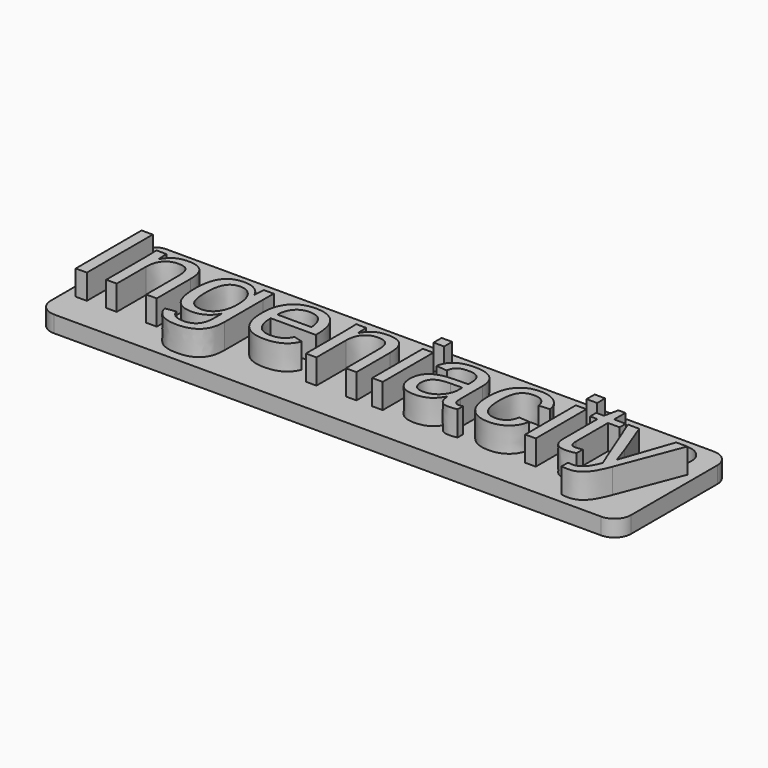
from build123d import *

# Parameters (mm, degrees)
F0_TEXT_SIZE = 14.4390369678
F1_DEPTH     = 3
F0_W         = 1.2701840333
F0_H         = 7.6278724981
F0_W_2       = 1.3468914172
F0_H_2       = 9.9336062139
F0_H_3       = 1.2137815451
F0_R         = 2
F2_DEPTH     = 2
F3_DEPTH     = 2


# Not quite as in the source:
# - Text() gives the source's letters only with a copy of the font that has no kerning and outlines rounded to 1/6400 em; it was checked with that copy


with BuildPart() as f1:
    # F0 (on Top) → F1 (new body)
    with BuildSketch(Plane.XY):
        with Locations((0, 4.1038933832)):
            Text('Ingeniacity', F0_TEXT_SIZE, font='Arimo', text_align=(TextAlign.LEFT, TextAlign.BOTTOM))
    extrude(amount=F1_DEPTH)


with BuildPart() as f2:
    # F0 (on Top) → F2 (new body)
    with BuildSketch(Plane.XY):
        with BuildLine():
            ThreePointArc((0, 2), (0.5857864376, 0.5857864376), (2, 0))
            Line((2, 0), (68, 0))
            ThreePointArc((68, 0), (69.4142135624, 0.5857864376), (70, 2))
            Line((70, 2), (70, 15))
            ThreePointArc((70, 15), (69.4142135624, 16.4142135624), (68, 17))
            Line((68, 17), (2, 17))
            ThreePointArc((2, 17), (0.5857864376, 16.4142135624), (0, 15))
            Line((0, 15), (0, 2))
        make_face()
        with BuildLine():
            Line((11.1045218681, 4.1038933832), (9.8275695362, 4.1038933832))
            Line((9.8275695362, 4.1038933832), (9.8275695362, 8.9409707674))
            add(Edge.make_bspline(
                [(9.8275695362, 8.9409707674), (9.8275695362, 9.6945080092), (9.6797950172, 10.1107583717)],
                knots=[0, 0, 0, 1, 1, 1], degree=2))
            add(Edge.make_bspline(
                [(9.6797950172, 10.1107583717), (9.5320204983, 10.5270087343), (9.2071421665, 10.709752796)],
                knots=[0, 0, 0, 1, 1, 1], degree=2))
            add(Edge.make_bspline(
                [(9.2071421665, 10.709752796), (8.8822638347, 10.8924968576), (8.2550681664, 10.8924968576)],
                knots=[0, 0, 0, 1, 1, 1], degree=2))
            add(Edge.make_bspline(
                [(8.2550681664, 10.8924968576), (7.3390917588, 10.8924968576), (6.8100364199, 10.2653011893)],
                knots=[0, 0, 0, 1, 1, 1], degree=2))
            add(Edge.make_bspline(
                [(6.8100364199, 10.2653011893), (6.280981081, 9.638105521), (6.280981081, 8.523592355)],
                knots=[0, 0, 0, 1, 1, 1], degree=2))
            Line((6.280981081, 8.523592355), (6.280981081, 4.1038933832))
            Line((6.280981081, 4.1038933832), (5.0130531473, 4.1038933832))
            Line((5.0130531473, 4.1038933832), (5.0130531473, 10.1028620234))
            add(Edge.make_bspline(
                [(5.0130531473, 10.1028620234), (5.0130531473, 11.4362168434), (4.9701872563, 11.7317658813)],
                knots=[0, 0, 0, 1, 1, 1], degree=2))
            Line((4.9701872563, 11.7317658813), (6.1681761047, 11.7317658813))
            add(Edge.make_bspline(
                [(6.1681761047, 11.7317658813), (6.1749444033, 11.6979243884), (6.1828407516, 11.5422535211)],
                knots=[0, 0, 0, 1, 1, 1], degree=2))
            add(Edge.make_bspline(
                [(6.1828407516, 11.5422535211), (6.1907370999, 11.3865826538), (6.2008895478, 11.185789796)],
                knots=[0, 0, 0, 1, 1, 1], degree=2))
            add(Edge.make_bspline(
                [(6.2008895478, 11.185789796), (6.2110419957, 10.9849969382), (6.2245785928, 10.4277403552)],
                knots=[0, 0, 0, 1, 1, 1], degree=2))
            Line((6.2245785928, 10.4277403552), (6.2471395881, 10.4277403552))
            add(Edge.make_bspline(
                [(6.2471395881, 10.4277403552), (6.6825667967, 11.2173751894), (7.2578721758, 11.5456376704)],
                knots=[0, 0, 0, 1, 1, 1], degree=2))
            add(Edge.make_bspline(
                [(7.2578721758, 11.5456376704), (7.833177555, 11.8739001515), (8.6859831759, 11.8739001515)],
                knots=[0, 0, 0, 1, 1, 1], degree=2))
            add(Edge.make_bspline(
                [(8.6859831759, 11.8739001515), (9.9403745125, 11.8739001515), (10.5224481903, 11.2500886325)],
                knots=[0, 0, 0, 1, 1, 1], degree=2))
            add(Edge.make_bspline(
                [(10.5224481903, 11.2500886325), (11.1045218681, 10.6262771135), (11.1045218681, 9.1868856158)],
                knots=[0, 0, 0, 1, 1, 1], degree=2))
            Line((11.1045218681, 9.1868856158), (11.1045218681, 4.1038933832))
        make_face(mode=Mode.SUBTRACT)
        with BuildLine():
            add(Edge.make_bspline(
                [(19.0978824894, 4.3227350372), (19.0978824894, 1.1077932124), (15.9055016598, 1.1077932124)],
                knots=[0, 0, 0, 1, 1, 1], degree=2))
            add(Edge.make_bspline(
                [(15.9055016598, 1.1077932124), (14.6556225223, 1.1077932124), (13.9156218777, 1.5973668096)],
                knots=[0, 0, 0, 1, 1, 1], degree=2))
            add(Edge.make_bspline(
                [(13.9156218777, 1.5973668096), (13.1756212331, 2.0869404067), (12.9635478777, 2.9893802172)],
                knots=[0, 0, 0, 1, 1, 1], degree=2))
            Line((12.9635478777, 2.9893802172), (14.2405002095, 3.1721242789))
            add(Edge.make_bspline(
                [(14.2405002095, 3.1721242789), (14.366841783, 2.6441969897), (14.8011409418, 2.3588003997)],
                knots=[0, 0, 0, 1, 1, 1], degree=2))
            add(Edge.make_bspline(
                [(14.8011409418, 2.3588003997), (15.2354401006, 2.0734038096), (15.9393431527, 2.0734038096)],
                knots=[0, 0, 0, 1, 1, 1], degree=2))
            add(Edge.make_bspline(
                [(15.9393431527, 2.0734038096), (17.8367228543, 2.0734038096), (17.8367228543, 4.2934057434)],
                knots=[0, 0, 0, 1, 1, 1], degree=2))
            Line((17.8367228543, 4.2934057434), (17.8367228543, 5.5207238856))
            Line((17.8367228543, 5.5207238856), (17.8231862571, 5.5207238856))
            add(Edge.make_bspline(
                [(17.8231862571, 5.5207238856), (17.4622103329, 4.7874915396), (16.8350146646, 4.4174912173)],
                knots=[0, 0, 0, 1, 1, 1], degree=2))
            add(Edge.make_bspline(
                [(16.8350146646, 4.4174912173), (16.2078189964, 4.047490895), (15.3685499726, 4.047490895)],
                knots=[0, 0, 0, 1, 1, 1], degree=2))
            add(Edge.make_bspline(
                [(15.3685499726, 4.047490895), (13.9652560673, 4.047490895), (13.3064750056, 4.9781319496)],
                knots=[0, 0, 0, 1, 1, 1], degree=2))
            add(Edge.make_bspline(
                [(13.3064750056, 4.9781319496), (12.647693944, 5.9087730042), (12.647693944, 7.9031649853)],
                knots=[0, 0, 0, 1, 1, 1], degree=2))
            add(Edge.make_bspline(
                [(12.647693944, 7.9031649853), (12.647693944, 9.9268862604), (13.3561091952, 10.8891127083)],
                knots=[0, 0, 0, 1, 1, 1], degree=2))
            add(Edge.make_bspline(
                [(13.3561091952, 10.8891127083), (14.0645244464, 11.8513391562), (15.5106842428, 11.8513391562)],
                knots=[0, 0, 0, 1, 1, 1], degree=2))
            add(Edge.make_bspline(
                [(15.5106842428, 11.8513391562), (16.3206239727, 11.8513391562), (16.9162342476, 11.4813388339)],
                knots=[0, 0, 0, 1, 1, 1], degree=2))
            add(Edge.make_bspline(
                [(16.9162342476, 11.4813388339), (17.5118445225, 11.1113385116), (17.8367228543, 10.4277403552)],
                knots=[0, 0, 0, 1, 1, 1], degree=2))
            Line((17.8367228543, 10.4277403552), (17.8502594514, 10.4277403552))
            add(Edge.make_bspline(
                [(17.8502594514, 10.4277403552), (17.8502594514, 10.6398137106), (17.8784606955, 11.1609727012)],
                knots=[0, 0, 0, 1, 1, 1], degree=2))
            add(Edge.make_bspline(
                [(17.8784606955, 11.1609727012), (17.9066619396, 11.6821316918), (17.9359912334, 11.7317658813)],
                knots=[0, 0, 0, 1, 1, 1], degree=2))
            Line((17.9359912334, 11.7317658813), (19.1407483804, 11.7317658813))
            add(Edge.make_bspline(
                [(19.1407483804, 11.7317658813), (19.0978824894, 11.3527411609), (19.0978824894, 10.152496213)],
                knots=[0, 0, 0, 1, 1, 1], degree=2))
            Line((19.0978824894, 10.152496213), (19.0978824894, 4.3227350372))
        make_face(mode=Mode.SUBTRACT)
        with BuildLine():
            Line((27.4589873336, 7.6504818384), (22.0172752764, 7.6504818384))
            add(Edge.make_bspline(
                [(22.0172752764, 7.6504818384), (22.0172752764, 6.3396880137), (22.5598672124, 5.6267605634)],
                knots=[0, 0, 0, 1, 1, 1], degree=2))
            add(Edge.make_bspline(
                [(22.5598672124, 5.6267605634), (23.1024591485, 4.9138331131), (24.1447771296, 4.9138331131)],
                knots=[0, 0, 0, 1, 1, 1], degree=2))
            add(Edge.make_bspline(
                [(24.1447771296, 4.9138331131), (24.9705095562, 4.9138331131), (25.4679795017, 5.2454797434)],
                knots=[0, 0, 0, 1, 1, 1], degree=2))
            add(Edge.make_bspline(
                [(25.4679795017, 5.2454797434), (25.9654494473, 5.5771263738), (26.1414252103, 6.0847487672)],
                knots=[0, 0, 0, 1, 1, 1], degree=2))
            Line((26.1414252103, 6.0847487672), (27.2536822767, 5.7688948335))
            add(Edge.make_bspline(
                [(27.2536822767, 5.7688948335), (26.5700841203, 3.961759113), (24.1447771296, 3.961759113)],
                knots=[0, 0, 0, 1, 1, 1], degree=2))
            add(Edge.make_bspline(
                [(24.1447771296, 3.961759113), (22.4527024849, 3.961759113), (21.5683114707, 4.9702356013)],
                knots=[0, 0, 0, 1, 1, 1], degree=2))
            add(Edge.make_bspline(
                [(21.5683114707, 4.9702356013), (20.6839204564, 5.9787120895), (20.6839204564, 7.9685918716)],
                knots=[0, 0, 0, 1, 1, 1], degree=2))
            add(Edge.make_bspline(
                [(20.6839204564, 7.9685918716), (20.6839204564, 9.856947175), (21.5683114707, 10.8654236633)],
                knots=[0, 0, 0, 1, 1, 1], degree=2))
            add(Edge.make_bspline(
                [(21.5683114707, 10.8654236633), (22.4527024849, 11.8739001515), (24.09514294, 11.8739001515)],
                knots=[0, 0, 0, 1, 1, 1], degree=2))
            add(Edge.make_bspline(
                [(24.09514294, 11.8739001515), (27.4589873336, 11.8739001515), (27.4589873336, 7.8196893029)],
                knots=[0, 0, 0, 1, 1, 1], degree=2))
            Line((27.4589873336, 7.8196893029), (27.4589873336, 7.6504818384))
        make_face(mode=Mode.SUBTRACT)
        with BuildLine():
            Line((35.1928965095, 4.1038933832), (33.9159441777, 4.1038933832))
            Line((33.9159441777, 4.1038933832), (33.9159441777, 8.9409707674))
            add(Edge.make_bspline(
                [(33.9159441777, 8.9409707674), (33.9159441777, 9.6945080092), (33.7681696587, 10.1107583717)],
                knots=[0, 0, 0, 1, 1, 1], degree=2))
            add(Edge.make_bspline(
                [(33.7681696587, 10.1107583717), (33.6203951397, 10.5270087343), (33.2955168079, 10.709752796)],
                knots=[0, 0, 0, 1, 1, 1], degree=2))
            add(Edge.make_bspline(
                [(33.2955168079, 10.709752796), (32.9706384762, 10.8924968576), (32.3434428079, 10.8924968576)],
                knots=[0, 0, 0, 1, 1, 1], degree=2))
            add(Edge.make_bspline(
                [(32.3434428079, 10.8924968576), (31.4274664002, 10.8924968576), (30.8984110613, 10.2653011893)],
                knots=[0, 0, 0, 1, 1, 1], degree=2))
            add(Edge.make_bspline(
                [(30.8984110613, 10.2653011893), (30.3693557224, 9.638105521), (30.3693557224, 8.523592355)],
                knots=[0, 0, 0, 1, 1, 1], degree=2))
            Line((30.3693557224, 8.523592355), (30.3693557224, 4.1038933832))
            Line((30.3693557224, 4.1038933832), (29.1014277887, 4.1038933832))
            Line((29.1014277887, 4.1038933832), (29.1014277887, 10.1028620234))
            add(Edge.make_bspline(
                [(29.1014277887, 10.1028620234), (29.1014277887, 11.4362168434), (29.0585618977, 11.7317658813)],
                knots=[0, 0, 0, 1, 1, 1], degree=2))
            Line((29.0585618977, 11.7317658813), (30.2565507461, 11.7317658813))
            add(Edge.make_bspline(
                [(30.2565507461, 11.7317658813), (30.2633190447, 11.6979243884), (30.271215393, 11.5422535211)],
                knots=[0, 0, 0, 1, 1, 1], degree=2))
            add(Edge.make_bspline(
                [(30.271215393, 11.5422535211), (30.2791117414, 11.3865826538), (30.2892641893, 11.185789796)],
                knots=[0, 0, 0, 1, 1, 1], degree=2))
            add(Edge.make_bspline(
                [(30.2892641893, 11.185789796), (30.2994166371, 10.9849969382), (30.3129532343, 10.4277403552)],
                knots=[0, 0, 0, 1, 1, 1], degree=2))
            Line((30.3129532343, 10.4277403552), (30.3355142295, 10.4277403552))
            add(Edge.make_bspline(
                [(30.3355142295, 10.4277403552), (30.7709414381, 11.2173751894), (31.3462468173, 11.5456376704)],
                knots=[0, 0, 0, 1, 1, 1], degree=2))
            add(Edge.make_bspline(
                [(31.3462468173, 11.5456376704), (31.9215521965, 11.8739001515), (32.7743578174, 11.8739001515)],
                knots=[0, 0, 0, 1, 1, 1], degree=2))
            add(Edge.make_bspline(
                [(32.7743578174, 11.8739001515), (34.028749154, 11.8739001515), (34.6108228317, 11.2500886325)],
                knots=[0, 0, 0, 1, 1, 1], degree=2))
            add(Edge.make_bspline(
                [(34.6108228317, 11.2500886325), (35.1928965095, 10.6262771135), (35.1928965095, 9.1868856158)],
                knots=[0, 0, 0, 1, 1, 1], degree=2))
            Line((35.1928965095, 9.1868856158), (35.1928965095, 4.1038933832))
        make_face(mode=Mode.SUBTRACT)
        with Locations((37.7298804267, 7.9178296323)):
            Rectangle(F0_W, F0_H, mode=Mode.SUBTRACT)
        with BuildLine():
            add(Edge.make_bspline(
                [(43.8247332968, 4.3249911368), (43.1794888323, 3.961759113), (42.2567441261, 3.961759113)],
                knots=[0, 0, 0, 1, 1, 1], degree=2))
            add(Edge.make_bspline(
                [(42.2567441261, 3.961759113), (41.1061333677, 3.961759113), (40.528571889, 4.5686498856)],
                knots=[0, 0, 0, 1, 1, 1], degree=2))
            add(Edge.make_bspline(
                [(40.528571889, 4.5686498856), (39.9510104103, 5.1755406581), (39.9510104103, 6.2336513359)],
                knots=[0, 0, 0, 1, 1, 1], degree=2))
            add(Edge.make_bspline(
                [(39.9510104103, 6.2336513359), (39.9510104103, 7.4181035872), (40.7304927966, 8.0520675541)],
                knots=[0, 0, 0, 1, 1, 1], degree=2))
            add(Edge.make_bspline(
                [(40.7304927966, 8.0520675541), (41.5099751829, 8.6860315209), (43.242659619, 8.7288974119)],
                knots=[0, 0, 0, 1, 1, 1], degree=2))
            Line((43.242659619, 8.7288974119), (44.957295259, 8.7582267058))
            Line((44.957295259, 8.7582267058), (44.957295259, 9.1733490186))
            add(Edge.make_bspline(
                [(44.957295259, 9.1733490186), (44.957295259, 10.1028620234), (44.5624778419, 10.5055757888)],
                knots=[0, 0, 0, 1, 1, 1], degree=2))
            add(Edge.make_bspline(
                [(44.5624778419, 10.5055757888), (44.1676604248, 10.9082895543), (43.3216231025, 10.9082895543)],
                knots=[0, 0, 0, 1, 1, 1], degree=2))
            add(Edge.make_bspline(
                [(43.3216231025, 10.9082895543), (42.4688174815, 10.9082895543), (42.080768363, 10.6183807651)],
                knots=[0, 0, 0, 1, 1, 1], degree=2))
            add(Edge.make_bspline(
                [(42.080768363, 10.6183807651), (41.6927192445, 10.328471976), (41.6137557611, 9.6945080092)],
                knots=[0, 0, 0, 1, 1, 1], degree=2))
            Line((41.6137557611, 9.6945080092), (40.2894253392, 9.814081284))
            add(Edge.make_bspline(
                [(40.2894253392, 9.814081284), (40.614303671, 11.8739001515), (43.3486962968, 11.8739001515)],
                knots=[0, 0, 0, 1, 1, 1], degree=2))
            add(Edge.make_bspline(
                [(43.3486962968, 11.8739001515), (44.7880877945, 11.8739001515), (45.5134237922, 11.2139910401)],
                knots=[0, 0, 0, 1, 1, 1], degree=2))
            add(Edge.make_bspline(
                [(45.5134237922, 11.2139910401), (46.2387597899, 10.5540819286), (46.2387597899, 9.3064588906)],
                knots=[0, 0, 0, 1, 1, 1], degree=2))
            Line((46.2387597899, 9.3064588906), (46.2387597899, 6.0215779805))
            add(Edge.make_bspline(
                [(46.2387597899, 6.0215779805), (46.2387597899, 5.4575530989), (46.3876623586, 5.1721565088)],
                knots=[0, 0, 0, 1, 1, 1], degree=2))
            add(Edge.make_bspline(
                [(46.3876623586, 5.1721565088), (46.5365649273, 4.8867599188), (46.9516872401, 4.8867599188)],
                knots=[0, 0, 0, 1, 1, 1], degree=2))
            add(Edge.make_bspline(
                [(46.9516872401, 4.8867599188), (47.1344313018, 4.8867599188), (47.366809553, 4.9363941084)],
                knots=[0, 0, 0, 1, 1, 1], degree=2))
            Line((47.366809553, 4.9363941084), (47.366809553, 4.1467592742))
            add(Edge.make_bspline(
                [(47.366809553, 4.1467592742), (46.8885164534, 4.0339542979), (46.3876623586, 4.0339542979)],
                knots=[0, 0, 0, 1, 1, 1], degree=2))
            add(Edge.make_bspline(
                [(46.3876623586, 4.0339542979), (45.6837593064, 4.0339542979), (45.3622651239, 4.4039546202)],
                knots=[0, 0, 0, 1, 1, 1], degree=2))
            add(Edge.make_bspline(
                [(45.3622651239, 4.4039546202), (45.0407709414, 4.7739549425), (44.9979050504, 5.5635897766)],
                knots=[0, 0, 0, 1, 1, 1], degree=2))
            Line((44.9979050504, 5.5635897766), (44.957295259, 5.5635897766))
            add(Edge.make_bspline(
                [(44.957295259, 5.5635897766), (44.4699777613, 4.6882231605), (43.8247332968, 4.3249911368)],
                knots=[0, 0, 0, 1, 1, 1], degree=2))
        make_face(mode=Mode.SUBTRACT)
        with BuildLine():
            add(Edge.make_bspline(
                [(49.7560189512, 10.2088987011), (49.304799046, 9.5388371418), (49.304799046, 7.9527991749)],
                knots=[0, 0, 0, 1, 1, 1], degree=2))
            add(Edge.make_bspline(
                [(49.304799046, 7.9527991749), (49.304799046, 6.4299319947), (49.7842201953, 5.6966996487)],
                knots=[0, 0, 0, 1, 1, 1], degree=2))
            add(Edge.make_bspline(
                [(49.7842201953, 5.6966996487), (50.2636413446, 4.9634673027), (51.2315080414, 4.9634673027)],
                knots=[0, 0, 0, 1, 1, 1], degree=2))
            add(Edge.make_bspline(
                [(51.2315080414, 4.9634673027), (51.9083378992, 4.9634673027), (52.3629419538, 5.3300834757)],
                knots=[0, 0, 0, 1, 1, 1], degree=2))
            add(Edge.make_bspline(
                [(52.3629419538, 5.3300834757), (52.8175460083, 5.6966996487), (52.923582686, 6.4592612886)],
                knots=[0, 0, 0, 1, 1, 1], degree=2))
            Line((52.923582686, 6.4592612886), (54.2050472169, 6.3735295066))
            add(Edge.make_bspline(
                [(54.2050472169, 6.3735295066), (54.0584007477, 5.2748090373), (53.2687659136, 4.6182840752)],
                knots=[0, 0, 0, 1, 1, 1], degree=2))
            add(Edge.make_bspline(
                [(53.2687659136, 4.6182840752), (52.4791310794, 3.961759113), (51.2653495343, 3.961759113)],
                knots=[0, 0, 0, 1, 1, 1], degree=2))
            add(Edge.make_bspline(
                [(51.2653495343, 3.961759113), (49.6657749702, 3.961759113), (48.8231217971, 4.9736197505)],
                knots=[0, 0, 0, 1, 1, 1], degree=2))
            add(Edge.make_bspline(
                [(48.8231217971, 4.9736197505), (47.9804686241, 5.985480388), (47.9804686241, 7.9257259806)],
                knots=[0, 0, 0, 1, 1, 1], degree=2))
            add(Edge.make_bspline(
                [(47.9804686241, 7.9257259806), (47.9804686241, 9.8501788765), (48.8265059464, 10.862039514)],
                knots=[0, 0, 0, 1, 1, 1], degree=2))
            add(Edge.make_bspline(
                [(48.8265059464, 10.862039514), (49.6725432688, 11.8739001515), (51.2518129371, 11.8739001515)],
                knots=[0, 0, 0, 1, 1, 1], degree=2))
            add(Edge.make_bspline(
                [(51.2518129371, 11.8739001515), (52.4227285912, 11.8739001515), (53.1943146292, 11.2670093789)],
                knots=[0, 0, 0, 1, 1, 1], degree=2))
            add(Edge.make_bspline(
                [(53.1943146292, 11.2670093789), (53.9659006672, 10.6601186064), (54.1644374255, 9.59523963)],
                knots=[0, 0, 0, 1, 1, 1], degree=2))
            Line((54.1644374255, 9.59523963), (52.8581557998, 9.4982273504))
            add(Edge.make_bspline(
                [(52.8581557998, 9.4982273504), (52.7611435202, 10.1321913172), (52.3584297547, 10.5055757888)],
                knots=[0, 0, 0, 1, 1, 1], degree=2))
            add(Edge.make_bspline(
                [(52.3584297547, 10.5055757888), (51.9557159893, 10.8789602604), (51.2157153447, 10.8789602604)],
                knots=[0, 0, 0, 1, 1, 1], degree=2))
            add(Edge.make_bspline(
                [(51.2157153447, 10.8789602604), (50.2072388565, 10.8789602604), (49.7560189512, 10.2088987011)],
                knots=[0, 0, 0, 1, 1, 1], degree=2))
        make_face(mode=Mode.SUBTRACT)
        with Locations((56.1870306507, 7.9178296323)):
            Rectangle(F0_W, F0_H, mode=Mode.SUBTRACT)
        with BuildLine():
            add(Edge.make_bspline(
                [(64.2774035517, 1.399958101), (63.7799336062, 1.1077932124), (63.1527379379, 1.1077932124)],
                knots=[0, 0, 0, 1, 1, 1], degree=2))
            add(Edge.make_bspline(
                [(63.1527379379, 1.1077932124), (62.6315789474, 1.1077932124), (62.2773713218, 1.1845005963)],
                knots=[0, 0, 0, 1, 1, 1], degree=2))
            Line((62.2773713218, 1.1845005963), (62.2773713218, 2.1365745963))
            add(Edge.make_bspline(
                [(62.2773713218, 2.1365745963), (62.5458471654, 2.0937087053), (62.8707254971, 2.0937087053)],
                knots=[0, 0, 0, 1, 1, 1], degree=2))
            add(Edge.make_bspline(
                [(62.8707254971, 2.0937087053), (64.0551777484, 2.0937087053), (64.7455442034, 3.8354175396)],
                knots=[0, 0, 0, 1, 1, 1], degree=2))
            Line((64.7455442034, 3.8354175396), (64.8651174783, 4.1399909756))
            Line((64.8651174783, 4.1399909756), (61.8419441132, 11.7317658813))
            Line((61.8419441132, 11.7317658813), (63.1956038289, 11.7317658813))
            Line((63.1956038289, 11.7317658813), (64.8019466916, 7.5173719664))
            add(Edge.make_bspline(
                [(64.8019466916, 7.5173719664), (64.838044284, 7.4181035872), (64.8876784736, 7.2804815161)],
                knots=[0, 0, 0, 1, 1, 1], degree=2))
            add(Edge.make_bspline(
                [(64.8876784736, 7.2804815161), (64.9373126632, 7.142859445), (65.204660457, 6.3599929094)],
                knots=[0, 0, 0, 1, 1, 1], degree=2))
            add(Edge.make_bspline(
                [(65.204660457, 6.3599929094), (65.4720082509, 5.5771263738), (65.4923131466, 5.4868823928)],
                knots=[0, 0, 0, 1, 1, 1], degree=2))
            Line((65.4923131466, 5.4868823928), (65.9863989429, 6.8743836014))
            Line((65.9863989429, 6.8743836014), (67.6581686918, 11.7317658813))
            Line((67.6581686918, 11.7317658813), (68.9982918104, 11.7317658813))
            Line((68.9982918104, 11.7317658813), (66.0653624263, 4.1038933832))
            add(Edge.make_bspline(
                [(66.0653624263, 4.1038933832), (65.5915815258, 2.8833435395), (65.1832275115, 2.2877332646)],
                knots=[0, 0, 0, 1, 1, 1], degree=2))
            add(Edge.make_bspline(
                [(65.1832275115, 2.2877332646), (64.7748734973, 1.6921229897), (64.2774035517, 1.399958101)],
                knots=[0, 0, 0, 1, 1, 1], degree=2))
        make_face(mode=Mode.SUBTRACT)
        with Locations((2.0068005286, 9.0706964902)):
            Rectangle(F0_W_2, F0_H_2, mode=Mode.SUBTRACT)
        with BuildLine():
            Line((61.699809843, 5.0988332742), (61.699809843, 4.1602958713))
            add(Edge.make_bspline(
                [(61.699809843, 4.1602958713), (61.0726141748, 3.9910884069), (60.4183453121, 3.9910884069)],
                knots=[0, 0, 0, 1, 1, 1], degree=2))
            add(Edge.make_bspline(
                [(60.4183453121, 3.9910884069), (58.8954781319, 3.9910884069), (58.8954781319, 5.719260644)],
                knots=[0, 0, 0, 1, 1, 1], degree=2))
            Line((58.8954781319, 5.719260644), (58.8954781319, 10.8090211751))
            Line((58.8954781319, 10.8090211751), (58.0133432172, 10.8090211751))
            Line((58.0133432172, 10.8090211751), (58.0133432172, 11.7317658813))
            Line((58.0133432172, 11.7317658813), (58.942856222, 11.7317658813))
            Line((58.942856222, 11.7317658813), (59.3173687434, 13.4396332227))
            Line((59.3173687434, 13.4396332227), (60.1634060657, 13.4396332227))
            Line((60.1634060657, 13.4396332227), (60.1634060657, 11.7317658813))
            Line((60.1634060657, 11.7317658813), (61.5734682696, 11.7317658813))
            Line((61.5734682696, 11.7317658813), (61.5734682696, 10.8090211751))
            Line((61.5734682696, 10.8090211751), (60.1634060657, 10.8090211751))
            Line((60.1634060657, 10.8090211751), (60.1634060657, 5.9945047862))
            add(Edge.make_bspline(
                [(60.1634060657, 5.9945047862), (60.1634060657, 5.4440165018), (60.342765978, 5.2217906984)],
                knots=[0, 0, 0, 1, 1, 1], degree=2))
            add(Edge.make_bspline(
                [(60.342765978, 5.2217906984), (60.5221258904, 4.9995648951), (60.966577497, 4.9995648951)],
                knots=[0, 0, 0, 1, 1, 1], degree=2))
            add(Edge.make_bspline(
                [(60.966577497, 4.9995648951), (61.2215167435, 4.9995648951), (61.699809843, 5.0988332742)],
                knots=[0, 0, 0, 1, 1, 1], degree=2))
        make_face(mode=Mode.SUBTRACT)
        with Locations((37.7298804267, 13.9607922132)):
            Rectangle(F0_W, F0_H_3, mode=Mode.SUBTRACT)
        with Locations((56.1870306507, 13.9607922132)):
            Rectangle(F0_W, F0_H_3, mode=Mode.SUBTRACT)
        with Locations((65.5549168587, 14.1784418374)):
            Circle(F0_R, mode=Mode.SUBTRACT)
    extrude(amount=-F2_DEPTH)


with BuildPart() as f3:
    # F0 (on Top) → F3 (new body)
    with BuildSketch(Plane.XY):
        with Locations((0, 4.1038933832)):
            Text('Ingeniacity', F0_TEXT_SIZE, font='Arimo', text_align=(TextAlign.LEFT, TextAlign.BOTTOM))
    extrude(amount=-F3_DEPTH)


solid = Compound([f1.part, f2.part, f3.part])
